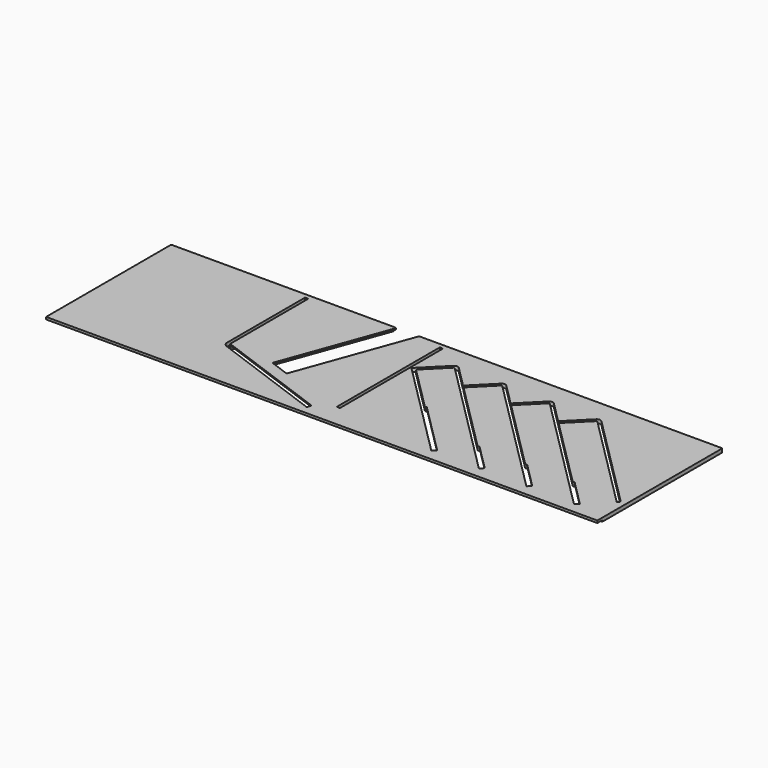
from build123d import *

# Parameters (mm, degrees)
F0_W     = 3.5
F0_H     = 140
F1_DEPTH = 4
F3_DEPTH = 2.5
F2_W     = 599.2343145751
F2_H     = 7
F4_DEPTH = 1.5


# Not quite as in the source:
# - a feature names something its author has since deleted; it is built from what else it names


with BuildPart() as f1:
    # F0 (on Top) → F1 (new body)
    with BuildSketch(Plane.XY):
        with BuildLine():
            Line((-299.8, -88.5), (299.4343145751, -88.5))
            Line((299.4343145751, -88.5), (299.4343145751, 80.5))
            ThreePointArc((299.4343145751, 80.5), (299.1414213562, 81.2071067812), (298.4343145751, 81.5))
            Line((298.4343145751, 81.5), (-29.5426009536, 81.5))
            ThreePointArc((-29.5426009536, 81.5), (-30.1161773899, 81.3191520443), (-30.4822935744, 80.8420201433))
            Line((-30.4822935744, 80.8420201433), (-32.577653202, 75.0850668809))
            Line((-32.577653202, 75.0850668809), (-74.9647554186, -41.3725393356))
            ThreePointArc((-74.9647554186, -41.3725393356), (-75.4818297777, -41.9368269793), (-76.2464681828, -41.9702118131))
            Line((-76.2464681828, -41.9702118131), (-95.9786819334, -34.7882733517))
            ThreePointArc((-95.9786819334, -34.7882733517), (-96.5429695771, -34.2711989926), (-96.5763544108, -33.5065605876))
            Line((-96.5763544108, -33.5065605876), (-55.2058449976, 80.1579798567))
            ThreePointArc((-55.2058449976, 80.1579798567), (-55.3263855741, 81.0735764364), (-56.1455376183, 81.5))
            Line((-56.1455376183, 81.5), (-175.9202302026, 81.5))
            Line((-175.9202302026, 81.5), (-202.5231668673, 81.5))
            Line((-202.5231668673, 81.5), (-298.8, 81.5))
            ThreePointArc((-298.8, 81.5), (-299.5071067812, 81.2071067812), (-299.8, 80.5))
            Line((-299.8, 80.5), (-299.8, -88.5))
        make_face()
        with BuildLine():
            ThreePointArc((182.4185499288, 56.2932249718), (185.2469770535, 57.4647978471), (188.0754041783, 56.2932249718))
            Line((188.0754041783, 56.2932249718), (293.4343145751, -49.0656854249))
            Line((293.4343145751, -49.0656854249), (290.9594408409, -51.5405591591))
            Line((290.9594408409, -51.5405591591), (185.9540838347, 53.4647978471))
            ThreePointArc((185.9540838347, 53.4647978471), (185.2469770535, 53.7576910659), (184.5398702723, 53.4647978471))
            Line((184.5398702723, 53.4647978471), (162.6195600555, 31.5444876303))
            ThreePointArc((162.6195600555, 31.5444876303), (162.3266668367, 30.8373808491), (162.6195600555, 30.1302740679))
            Line((162.6195600555, 30.1302740679), (238.6335390331, -45.8837049096))
            ThreePointArc((238.6335390331, -45.8837049096), (239.3406458143, -46.1765981284), (240.0477525955, -45.8837049096))
            Line((240.0477525955, -45.8837049096), (240.4013059861, -45.530151519))
            Line((240.4013059861, -45.530151519), (268.6855772335, -73.8144227665))
            Line((268.6855772335, -73.8144227665), (267.6249170617, -74.8750829383))
            Line((267.6249170617, -74.8750829383), (265.1500433276, -77.3499566724))
            Line((265.1500433276, -77.3499566724), (156.962705806, 30.8373808491))
            Line((156.962705806, 30.8373808491), (133.9817354175, 53.8183512377))
            ThreePointArc((133.9817354175, 53.8183512377), (133.2746286363, 54.1112444565), (132.5675218551, 53.8183512377))
            Line((132.5675218551, 53.8183512377), (110.6472116383, 31.8980410209))
            ThreePointArc((110.6472116383, 31.8980410209), (110.3543184195, 31.1909342397), (110.6472116383, 30.4838274585))
            Line((110.6472116383, 30.4838274585), (186.6611906159, -45.530151519))
            ThreePointArc((186.6611906159, -45.530151519), (187.3682973971, -45.8230447378), (188.0754041783, -45.530151519))
            Line((188.0754041783, -45.530151519), (188.4289575688, -45.1765981284))
            Line((188.4289575688, -45.1765981284), (216.7132288163, -73.4608693759))
            Line((216.7132288163, -73.4608693759), (215.6525686445, -74.5215295477))
            Line((215.6525686445, -74.5215295477), (213.1776949104, -76.9964032818))
            Line((213.1776949104, -76.9964032818), (104.9903573888, 31.1909342397))
            Line((104.9903573888, 31.1909342397), (82.0093870003, 54.1719046283))
            ThreePointArc((82.0093870003, 54.1719046283), (81.3022802191, 54.4647978471), (80.5951734379, 54.1719046283))
            Line((80.5951734379, 54.1719046283), (58.6748632211, 32.2515944115))
            ThreePointArc((58.6748632211, 32.2515944115), (58.3819700023, 31.5444876303), (58.6748632211, 30.8373808491))
            Line((58.6748632211, 30.8373808491), (134.6888421987, -45.1765981284))
            ThreePointArc((134.6888421987, -45.1765981284), (135.3959489799, -45.4694913472), (136.103055761, -45.1765981284))
            Line((136.103055761, -45.1765981284), (136.4566091516, -44.8230447378))
            Line((136.4566091516, -44.8230447378), (164.7408803991, -73.1073159853))
            Line((164.7408803991, -73.1073159853), (163.6802202273, -74.1679761571))
            Line((163.6802202273, -74.1679761571), (161.2053464932, -76.6428498912))
            Line((161.2053464932, -76.6428498912), (53.0180089716, 31.5444876303))
            Line((53.0180089716, 31.5444876303), (30.0370385831, 54.5254580189))
            ThreePointArc((30.0370385831, 54.5254580189), (29.3299318019, 54.8183512377), (28.6228250207, 54.5254580189))
            Line((28.6228250207, 54.5254580189), (6.7025148039, 32.6051478021))
            ThreePointArc((6.7025148039, 32.6051478021), (6.4096215851, 31.8980410209), (6.7025148039, 31.1909342397))
            Line((6.7025148039, 31.1909342397), (54.432222534, -16.5387734904))
            ThreePointArc((54.432222534, -16.5387734904), (55.1393293152, -16.8316667092), (55.8464360964, -16.5387734904))
            Line((55.8464360964, -16.5387734904), (56.199989487, -16.1852200998))
            Line((56.199989487, -16.1852200998), (112.7685319819, -72.7537625947))
            Line((112.7685319819, -72.7537625947), (111.7078718101, -73.8144227665))
            Line((111.7078718101, -73.8144227665), (109.232998076, -76.2892965006))
            Line((109.232998076, -76.2892965006), (1.0456605544, 31.8980410209))
            Line((1.0456605544, 31.8980410209), (26.5015046771, 57.3538851436))
            ThreePointArc((26.5015046771, 57.3538851436), (29.3299318019, 58.5254580189), (32.1583589266, 57.3538851436))
            Line((32.1583589266, 57.3538851436), (55.4928827058, 34.0193613645))
            Line((55.4928827058, 34.0193613645), (78.4738530943, 57.000331753))
            ThreePointArc((78.4738530943, 57.000331753), (81.3022802191, 58.1719046283), (84.1307073438, 57.000331753))
            Line((84.1307073438, 57.000331753), (107.465231123, 33.6658079739))
            Line((107.465231123, 33.6658079739), (130.4462015116, 56.6467783624))
            ThreePointArc((130.4462015116, 56.6467783624), (133.2746286363, 57.8183512377), (136.103055761, 56.6467783624))
            Line((136.103055761, 56.6467783624), (159.4375795402, 33.3122545833))
            Line((159.4375795402, 33.3122545833), (182.4185499288, 56.2932249718))
        make_face(mode=Mode.SUBTRACT)
        with BuildLine():
            Line((-150.3, -29.2987547707), (-150.3, 76.504496433))
            Line((-150.3, 76.504496433), (-146.8, 76.504496433))
            Line((-146.8, 76.504496433), (-146.8, -29.0886925093))
            ThreePointArc((-146.8, -29.0886925093), (-146.2574561329, -30.8094218183), (-144.82606043, -31.9077703716))
            Line((-144.82606043, -31.9077703716), (-144.313030215, -30.4982314405))
            Line((-144.313030215, -30.4982314405), (-101.0871696588, -46.2311580334))
            Line((-101.0871696588, -46.2311580334), (-69.1376205521, -57.8598429065))
            Line((-69.1376205521, -57.8598429065), (-22.2894341652, -74.9111882807))
            Line((-22.2894341652, -74.9111882807), (-22.2894341652, -76.5074549394))
            Line((-22.2894341652, -76.5074549394), (-23.4865046669, -79.7963791122))
            Line((-23.4865046669, -79.7963791122), (-146.3577922078, -34.9348430622))
            ThreePointArc((-146.3577922078, -34.9348430622), (-149.2166428204, -32.7377405771), (-150.3, -29.2987547707))
        make_face(mode=Mode.SUBTRACT)
        with Locations((-2.05, 6.5)):
            Rectangle(F0_W, F0_H, mode=Mode.SUBTRACT)
    extrude(amount=F1_DEPTH)

    # F2 (on face) → F3 (cut)
    with BuildSketch(Plane(origin=(0, 0, 0), x_dir=(1, 0, 0), z_dir=(0, 0, -1))):
        Polygon((275.7566450454, 66.7433549546), (268.6855772335, 73.8144227665), (240.4013059861, 45.530151519), (247.4723737979, 38.4590837072), align=None)
        Polygon((216.7132288163, 73.4608693759), (188.4289575688, 45.1765981284), (195.5000253807, 38.1055303166), (223.7842966282, 66.389801564), align=None)
        Polygon((164.7408803991, 73.1073159853), (136.4566091516, 44.8230447378), (143.5276769635, 37.751976926), (171.811948211, 66.0362481734), align=None)
        Polygon((119.8395997938, 65.6826947828), (112.7685319819, 72.7537625947), (56.199989487, 16.1852200998), (63.2710572988, 9.1141522879), align=None)
        with BuildLine():
            Line((-56.1455376183, -81.5), (-57.5446454063, -81.5))
            Line((-57.5446454063, -81.5), (-55.4138746932, -87.3542444202))
            Line((-55.4138746932, -87.3542444202), (-52.4068583067, -86.2597799616))
            Line((-52.4068583067, -86.2597799616), (-95.9935465755, 33.3700433199))
            Line((-95.9935465755, 33.3700433199), (-75.1543020742, 41.3004074501))
            Line((-75.1543020742, 41.3004074501), (-28.7703498409, -86.1384539359))
            Line((-28.7703498409, -86.1384539359), (-28.5940280937, -86.0677343446))
            Line((-28.5940280937, -86.0677343446), (-25.5870117072, -84.9732698859))
            Line((-25.5870117072, -84.9732698859), (-26.8511785612, -81.5))
            Line((-26.8511785612, -81.5), (-29.5426009536, -81.5))
            ThreePointArc((-29.5426009536, -81.5), (-30.1161773899, -81.3191520443), (-30.4822935744, -80.8420201433))
            Line((-30.4822935744, -80.8420201433), (-74.9647554186, 41.3725393356))
            ThreePointArc((-74.9647554186, 41.3725393356), (-75.4818297777, 41.9368269793), (-76.2464681828, 41.9702118131))
            Line((-76.2464681828, 41.9702118131), (-95.9786819334, 34.7882733517))
            ThreePointArc((-95.9786819334, 34.7882733517), (-96.5429695771, 34.2711989926), (-96.5763544108, 33.5065605876))
            Line((-96.5763544108, 33.5065605876), (-55.2058449976, -80.1579798567))
            ThreePointArc((-55.2058449976, -80.1579798567), (-55.3263855741, -81.0735764364), (-56.1455376183, -81.5))
        make_face()
        with BuildLine():
            Line((-100.2390988931, 35.8020468909), (-57.5446454063, -81.5))
            Line((-57.5446454063, -81.5), (-56.1455376183, -81.5))
            ThreePointArc((-56.1455376183, -81.5), (-55.3263855741, -81.0735764364), (-55.2058449976, -80.1579798567))
            Line((-55.2058449976, -80.1579798567), (-96.5763544108, 33.5065605876))
            ThreePointArc((-96.5763544108, 33.5065605876), (-96.5429695771, 34.2711989926), (-95.9786819334, 34.7882733517))
            Line((-95.9786819334, 34.7882733517), (-76.2464681828, 41.9702118131))
            ThreePointArc((-76.2464681828, 41.9702118131), (-75.4818297777, 41.9368269793), (-74.9647554186, 41.3725393356))
            Line((-74.9647554186, 41.3725393356), (-30.4822935744, -80.8420201433))
            ThreePointArc((-30.4822935744, -80.8420201433), (-30.1161773899, -81.3191520443), (-29.5426009536, -81.5))
            Line((-29.5426009536, -81.5), (-26.8511785612, -81.5))
            Line((-26.8511785612, -81.5), (-73.1360856122, 45.666736984))
            Line((-73.1360856122, 45.666736984), (-18.1429199874, 65.6826123595))
            Line((-18.1429199874, 65.6826123595), (-21.7011533658, 75.5613879342))
            Line((-21.7011533658, 75.5613879342), (-22.2894341652, 75.3472712338))
            Line((-22.2894341652, 75.3472712338), (-22.2894341652, 74.9111882807))
            Line((-22.2894341652, 74.9111882807), (-143.8418430652, 30.6697295378))
            Line((-143.8418430652, 30.6697295378), (-140.3907859198, 21.1880279576))
            Line((-140.3907859198, 21.1880279576), (-100.2390988931, 35.8020468909))
        make_face()
    extrude(amount=-F3_DEPTH, mode=Mode.SUBTRACT)

    # F2 (on face) → F4 (cut)
    with BuildSketch(Plane(origin=(0, 0, 0), x_dir=(1, 0, 0), z_dir=(0, 0, -1))):
        with Locations((-0.1828427125, 85)):
            Rectangle(F2_W, F2_H)
    extrude(amount=-F4_DEPTH, mode=Mode.SUBTRACT)


solid = f1.part
